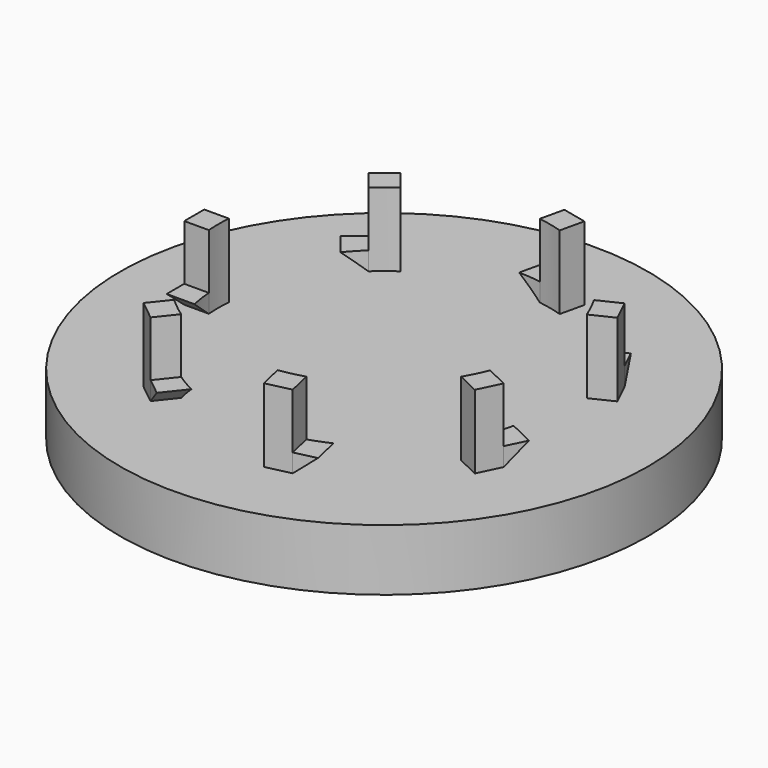
from build123d import *

# Parameters (mm, degrees)
F0_R            = 21.5
F0_R_2          = 13.5
F1_DEPTH        = 5
F3_DEPTH        = 6
F4_R            = 3.325
F5_DEPTH        = 4.5
F7_END_RADIUS   = 13.5
F7_REACH        = 39.2960714607
F7_COPIES_COUNT = 7


# Not quite as in the source:
# - a pattern or mirror of a feature is missing from the dataset's text; its kind, count and spacing are read off the source's solid


with BuildPart() as f1:
    # F0 (on Top) → F1 (new body)
    with BuildSketch(Plane.XY):
        Circle(F0_R)
        Circle(F0_R_2, mode=Mode.SUBTRACT)
        Circle(F0_R_2)
    extrude(amount=F1_DEPTH)

    # F2 (on face) → F3 (join)
    with BuildSketch(Plane.XY.offset(5)):
        with BuildLine():
            ThreePointArc((-13.4614857204, -1.0190202158), (-13.5, 0), (-13.4614857204, 1.0190202158))
            Line((-13.4614857204, 1.0190202158), (-15.4614857204, 1.0190202158))
            Line((-15.4614857204, 1.0190202158), (-15.4614857204, -1.0190202158))
            Line((-15.4614857204, -1.0190202158), (-13.4614857204, -1.0190202158))
        make_face()
        with BuildLine():
            ThreePointArc((-7.5963969786, -11.1599620494), (-8.4171123251, -10.5547250133), (-9.1898011505, -9.8892646246))
            Line((-9.1898011505, -9.8892646246), (-10.4367807542, -11.4529275895))
            Line((-10.4367807542, -11.4529275895), (-8.8433765823, -12.7236250143))
            Line((-8.8433765823, -12.7236250143), (-7.5963969786, -11.1599620494))
        make_face()
        with BuildLine():
            ThreePointArc((3.9889336264, -12.8972248381), (3.0040326084, -13.1615268145), (2.0019911235, -13.3507314984))
            Line((2.0019911235, -13.3507314984), (2.4470329914, -15.3005873227))
            Line((2.4470329914, -15.3005873227), (4.4339754943, -14.8470806625))
            Line((4.4339754943, -14.8470806625), (3.9889336264, -12.8972248381))
        make_face()
        with BuildLine():
            ThreePointArc((12.5705158512, -4.9226142683), (12.1630797167, -5.8574304781), (11.6862432483, -6.7588252486))
            Line((11.6862432483, -6.7588252486), (13.4881809841, -7.6265927268))
            Line((13.4881809841, -7.6265927268), (14.372453587, -5.7903817465))
            Line((14.372453587, -5.7903817465), (12.5705158512, -4.9226142683))
        make_face()
        with BuildLine():
            ThreePointArc((11.6862432483, 6.7588252486), (12.1630797167, 5.8574304781), (12.5705158512, 4.9226142683))
            Line((12.5705158512, 4.9226142683), (14.372453587, 5.7903817465))
            Line((14.372453587, 5.7903817465), (13.4881809841, 7.6265927268))
            Line((13.4881809841, 7.6265927268), (11.6862432483, 6.7588252486))
        make_face()
        with BuildLine():
            ThreePointArc((2.0019911235, 13.3507314984), (3.0040326084, 13.1615268145), (3.9889336264, 12.8972248381))
            Line((3.9889336264, 12.8972248381), (4.4339754943, 14.8470806625))
            Line((4.4339754943, 14.8470806625), (2.4470329914, 15.3005873227))
            Line((2.4470329914, 15.3005873227), (2.0019911235, 13.3507314984))
        make_face()
        with BuildLine():
            ThreePointArc((-9.1898011505, 9.8892646246), (-8.4171123251, 10.5547250133), (-7.5963969786, 11.1599620494))
            Line((-7.5963969786, 11.1599620494), (-8.8433765823, 12.7236250143))
            Line((-8.8433765823, 12.7236250143), (-10.4367807542, 11.4529275895))
            Line((-10.4367807542, 11.4529275895), (-9.1898011505, 9.8892646246))
        make_face()
    extrude(amount=F3_DEPTH)

    # F4 (on face) → F5 (cut)
    with BuildSketch(Plane(origin=(0, 0, 0), x_dir=(1, 0, 0), z_dir=(0, 0, -1))):
        with Locations((-17.5, 0)):
            Circle(F4_R)
        with Locations((17.5, 0)):
            Circle(F4_R)
    extrude(amount=-F5_DEPTH, mode=Mode.SUBTRACT)

    f7_end = (Plane(origin=(0, 0, 8), x_dir=(-1, 0, 0), z_dir=(0, 0, -1)) * Cylinder(F7_END_RADIUS, 202.1882593652, mode=Mode.PRIVATE)).faces().sort_by_distance((-13.5, 0, 8))[0]
    # F6 (on face) → F7 (join, up to the whole of a round face its end follows)
    with BuildSketch(Plane(origin=(-15.4614857204, 0, 0), x_dir=(0, -1, 0), z_dir=(-1, 0, 0))):
        Polygon((1.0190202158, 6.5), (1.0190202158, 5), (2.8066506047, 6.5), align=None)
    f7_long = extrude(amount=-F7_REACH, mode=Mode.PRIVATE)
    f7 = split(f7_long, bisect_by=f7_end, keep=Keep.ALL, mode=Mode.PRIVATE).solids().sort_by_distance((-15.4614857204, -1.6148970121, 6))[0]
    add(f7)

    # F7_copies: F7 ×7 about axis
    f7_copies_axis = Axis((0, 0, 0), (0, 0, 1))
    for i in range(1, F7_COPIES_COUNT):
        add(f7.rotate(f7_copies_axis, i * 360 / F7_COPIES_COUNT))


solid = f1.part
